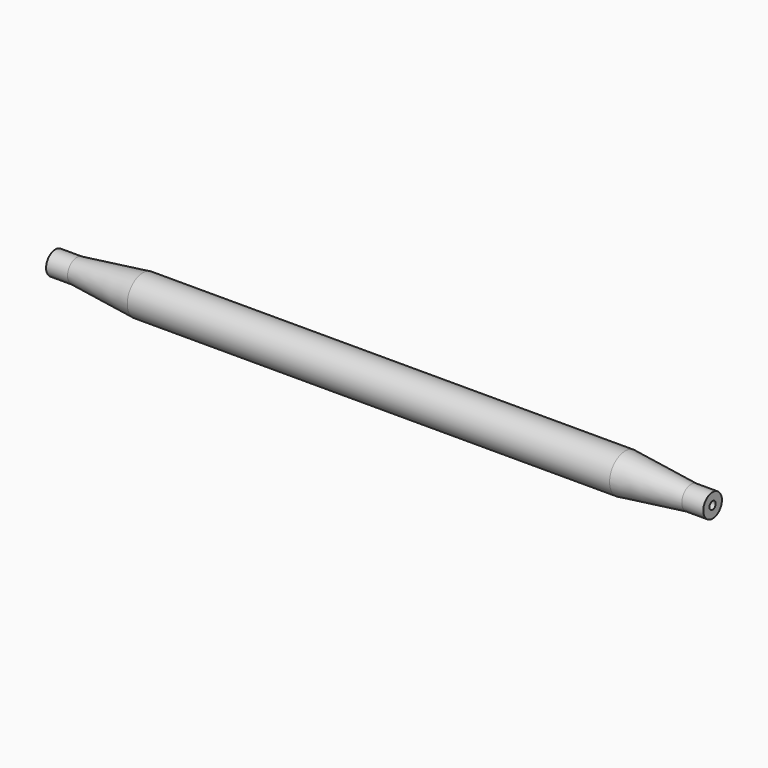
from build123d import *

# Parameters (mm, degrees)
F0_R       = 31.75
F1_DEPTH   = 393.7
F3_R       = 19.05
F4_DEPTH   = 35.052
F1_FACE_R  = 31.75
F4_FACE_R  = 19.05
F1_FACE1_R = 31.75
F5_FACE_R  = 19.05
F9_D       = 12.7
F9_DEPTH   = 44.45
F9_TIP     = 3.8154649308
F11_D      = 12.7
F11_DEPTH  = 44.45
F11_TIP    = 3.8154649308


with BuildPart() as f1:
    # F0 (on Right) → F1 (new body, symmetric)
    with BuildSketch(Plane.YZ):
        Circle(F0_R)
    extrude(amount=F1_DEPTH, both=True)



with BuildPart() as f4:
    # F3 (on offset) → F4 (new body)
    with BuildSketch(Plane.YZ.offset(536.448)):
        Circle(F3_R)
    extrude(amount=-F4_DEPTH)


with BuildPart() as f5_1:
    # F5: instance of F4
    add(f4.part.mirror(Plane.YZ))


with BuildPart() as f1_1:
    add(f1.part)

    add(f4.part)  # F6 merges F4
    # F1_face (on face) → F6 section 0
    with BuildSketch(Plane.YZ.offset(393.7)):
        Circle(F1_FACE_R)
    # F4_face (on face) → F6 section 1
    with BuildSketch(Plane(origin=(501.396, 0, 0), x_dir=(0, 1, 0), z_dir=(-1, 0, 0))):
        Circle(F4_FACE_R)
    loft()


    add(f5_1.part)  # F7 merges F5_1
    # F1_face1 (on face) → F7 section 0
    with BuildSketch(Plane(origin=(-393.7, 0, 0), x_dir=(0, 1, 0), z_dir=(-1, 0, 0))):
        Circle(F1_FACE1_R)
    # F5_face (on face) → F7 section 1
    with BuildSketch(Plane.YZ.offset(-501.396)):
        Circle(F5_FACE_R)
    loft()

    # F9
    with Locations(Plane.YZ.offset(536.448)):
        with Locations((0, 0)):
            Hole(F9_D / 2, depth=F9_DEPTH)
            with Locations((0, 0, -(F9_DEPTH + F9_TIP / 2))):  # 118° drill point
                Cone(0, F9_D / 2, F9_TIP, mode=Mode.SUBTRACT)

    # F11
    with Locations(Plane(origin=(-536.448, 0, 0), x_dir=(0, -1, 0), z_dir=(-1, 0, 0))):
        with Locations((0, 0)):
            Hole(F11_D / 2, depth=F11_DEPTH)
            with Locations((0, 0, -(F11_DEPTH + F11_TIP / 2))):  # 118° drill point
                Cone(0, F11_D / 2, F11_TIP, mode=Mode.SUBTRACT)


solid = f1_1.part
